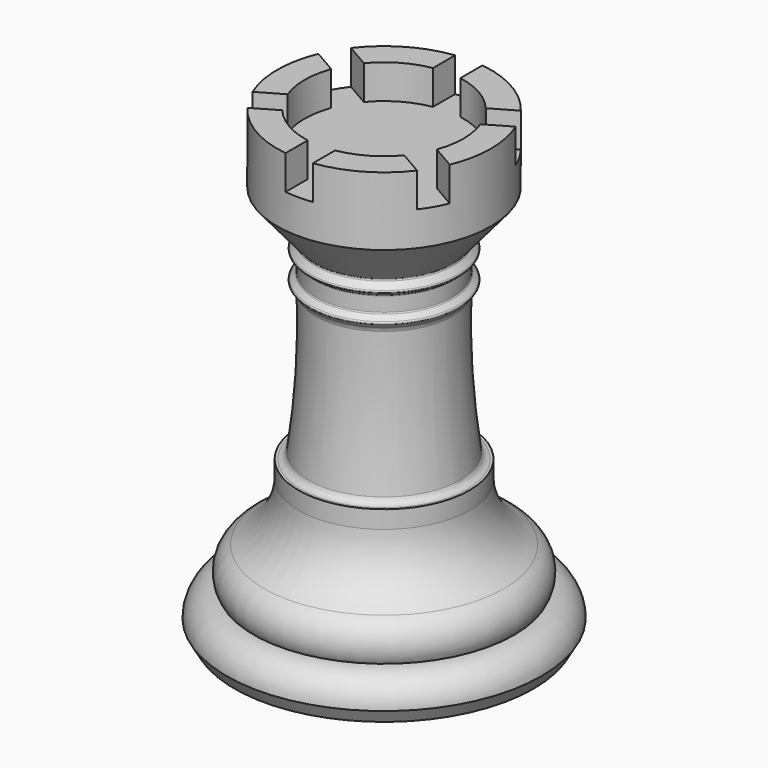
from build123d import *

# Parameters (mm, degrees)
F2_R            = 0.8
F3_R            = 0.2
F6_W            = 3.2
F6_H            = 4
F7_DEPTH        = 25
F7_COPIES_COUNT = 6


# Not quite as in the source:
# - a pattern or mirror of a feature is missing from the dataset's text; its kind, count and spacing are read off the source's solid


with BuildPart() as f1:
    # F0 (on Front) → F1 (revolve)
    with BuildSketch(Plane.XZ):
        with BuildLine():
            Line((0, 50), (0, 0))
            Line((0, 0), (17.5, 0))
            Line((17.5, 0), (18.4237604307, 1.6))
            ThreePointArc((18.4237604307, 1.6), (17.4865021305, 3.8627416998), (15.2237604307, 4.8))
            ThreePointArc((15.2237604307, 4.8), (15.5410710466, 7.2370185337), (14.0366718336, 9.180347731))
            ThreePointArc((14.0366718336, 9.180347731), (11.134597803, 12.0196080875), (10, 15.9178283066))
            Line((10, 15.9178283066), (10, 18))
            Line((10, 18), (9, 18))
            ThreePointArc((9, 18), (8.0941169003, 26.7419983148), (8, 35.5303030852))
            Line((8, 35.5303030852), (8.8, 36.4837059593))
            Line((8.8, 36.4837059593), (8, 37.1549856642))
            Line((8, 37.1549856642), (8, 39.0124262543))
            Line((8, 39.0124262543), (8.8, 39.6837059593))
            Line((8.8, 39.6837059593), (8, 40.6371088333))
            Line((8, 40.6371088333), (12.5, 46))
            Line((12.5, 46), (12.5, 54))
            Line((12.5, 54), (9.3, 54))
            Line((9.3, 54), (9.3, 50))
            Line((9.3, 50), (3.2, 50))
            Line((3.2, 50), (0, 50))
        make_face()
    revolve(axis=Axis((0, 0, 47.5), (0, 0, 1)))

    # F2
    f2_edges = [f1.edges().sort_by_distance(p)[0] for p in [
        (-8, 0, 35.530303),
        (-9, 0, 18),
    ]]
    fillet(f2_edges, radius=F2_R)

    # F3
    f3_edges = [f1.edges().sort_by_distance(p)[0] for p in [
        (-8.8, 0, 39.683706),
        (-8.8, 0, 36.483706),
        (-8, 0, 39.012426),
        (-8, 0, 37.154986),
        (-8, 0, 40.637109),
    ]]
    fillet(f3_edges, radius=F3_R)

    # F4 (on Front) → F5 (revolve, cut)
    with BuildSketch(Plane.XZ):
        with BuildLine():
            ThreePointArc((0, 18), (1.767766953, 18.732233047), (2.5, 20.5))
            Line((2.5, 20.5), (2.5, 35.5))
            ThreePointArc((2.5, 35.5), (1.767766953, 37.267766953), (0, 38))
            Line((0, 38), (0, 18))
        make_face()
    revolve(axis=Axis((0, 0, 28), (0, 0, -1)), mode=Mode.SUBTRACT)

    # F6 (on Front) → F7 (cut)
    with BuildSketch(Plane.XZ):
        with Locations((0, 52)):
            Rectangle(F6_W, F6_H)
    f7 = extrude(amount=-F7_DEPTH, mode=Mode.SUBTRACT)

    # F7_copies: F7 ×6 about axis
    f7_copies_axis = Axis((0, 0, 0), (0, 0, 1))
    for i in range(1, F7_COPIES_COUNT):
        add(f7.rotate(f7_copies_axis, i * 360 / F7_COPIES_COUNT), mode=Mode.SUBTRACT)


solid = f1.part
